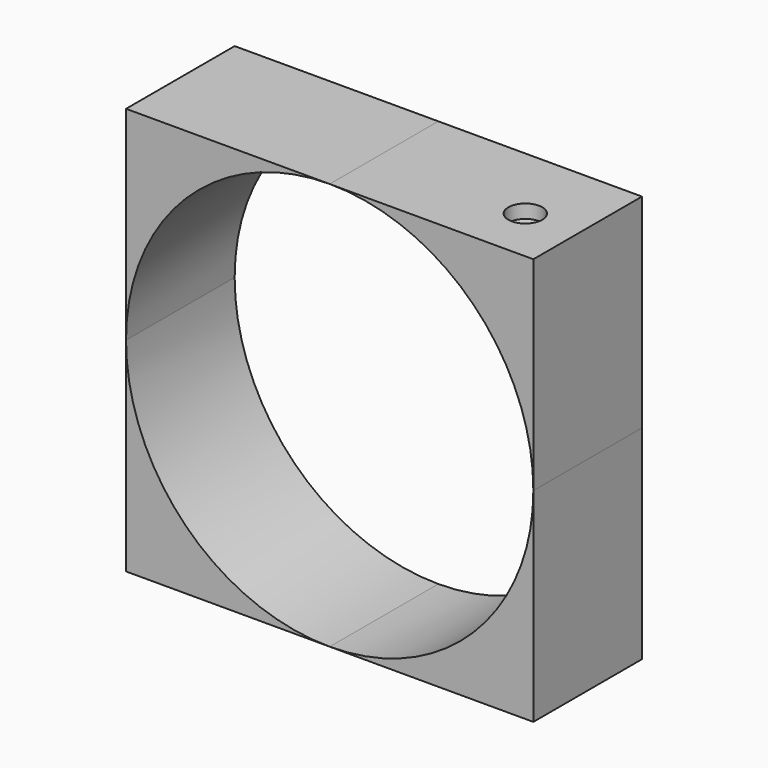
from build123d import *

# Parameters (mm, degrees)
F0_W     = 76.2
F0_H     = 76.2
F1_DEPTH = 25.4
F3_DEPTH = 25.4
F4_T     = -2.54
F6_D     = 6.35


# Not quite as in the source:
# - a shell that OpenCascade refuses in one call is made with other operations: the cavity is built on its own and cut out


with BuildPart() as f1:
    # F0 (on Front) → F1 (new body)
    with BuildSketch(Plane.XZ):
        Rectangle(F0_W, F0_H)
    extrude(amount=F1_DEPTH)

    # F2 (on face) → F3 (cut)
    with BuildSketch(Plane.XZ.offset(25.4)):
        with BuildLine():
            ThreePointArc((0, -38.1), (26.9407683632, -26.9407683632), (38.1, 0))
            ThreePointArc((38.1, 0), (26.9407683632, 26.9407683632), (0, 38.1))
            ThreePointArc((0, 38.1), (-26.9407683632, 26.9407683632), (-38.1, 0))
            ThreePointArc((-38.1, 0), (-26.9407683632, -26.9407683632), (0, -38.1))
        make_face()
    extrude(amount=-F3_DEPTH, mode=Mode.SUBTRACT)

    # F4: a shell. OpenCascade refuses it in one call, so the cavity is built on its own and cut out:
    # the body offset inwards by the wall thickness, plus a prism from it out through each open face.
    f4_core = offset(f1.part, amount=F4_T, mode=Mode.PRIVATE)
    f4_exits = [f4_core.faces().sort_by_distance(p)[0] for p in [
        (30.776271, -2.54, 30.776271),
        (-30.776271, -2.54, 30.776271),
        (-30.776271, -2.54, -30.776271),
        (30.776271, -2.54, -30.776271),
    ]]
    add(f4_core, mode=Mode.SUBTRACT)
    extrude(f4_exits, amount=-F4_T, mode=Mode.SUBTRACT)

    # F6 (through all)
    with Locations(Plane.XY.offset(38.1)):
        with Locations((28.1502772123, -14.8352207616)):
            Hole(F6_D / 2)


solid = f1.part
